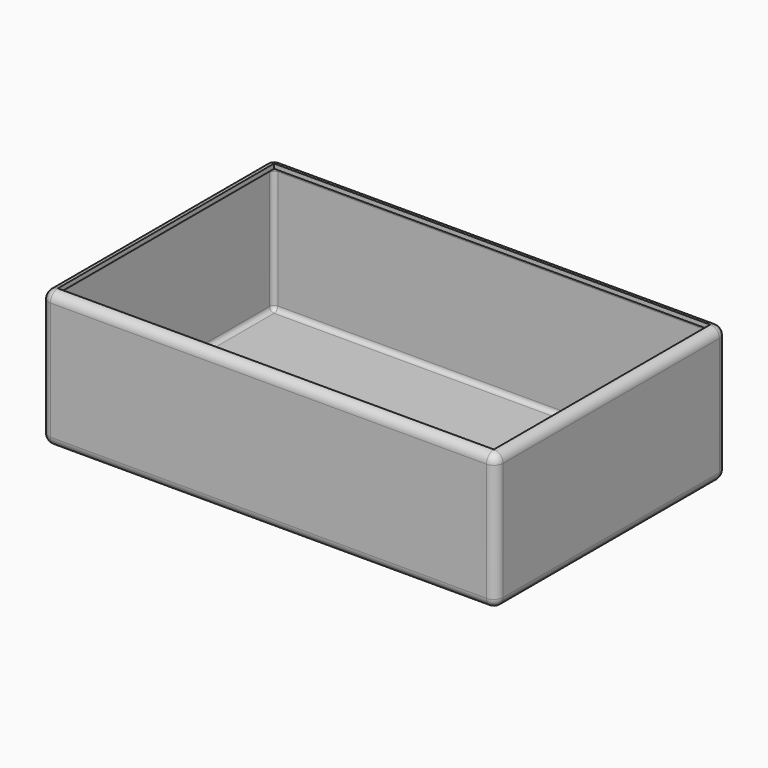
from build123d import *

# Parameters (mm, degrees)
F0_W     = 155.229896307
F0_H     = 82.4026092887
F1_DEPTH = 75.438
F2_DEPTH = 77.216
F3_DEPTH = 96.012
F4_R     = 5.08
F5_T     = -2.54
F6_R     = 16.8009840587
F7_DEPTH = 2.54


# Not quite as in the source:
# - a shell that OpenCascade refuses in one call is made with other operations: the cavity is built on its own and cut out


with BuildPart() as f1:
    # F0 (on Top) → F1 (new body)
    with BuildSketch(Plane.XY):
        with Locations((77.6149481535, 41.2013046443)):
            Rectangle(F0_W, F0_H)
    extrude(amount=F1_DEPTH)

    # F2 (add): a face of the model
    f2_faces = [f1.faces().sort_by_distance(p)[0] for p in [
        (77.6149481535, 0, 37.719),
    ]]
    extrude(f2_faces, amount=F2_DEPTH)

    # F3 (add): a face of the model
    f3_faces = [f1.faces().sort_by_distance(p)[0] for p in [
        (0, 2.5933046443, 37.719),
    ]]
    extrude(f3_faces, amount=F3_DEPTH)

    # F4
    f4_edges = [f1.edges().sort_by_distance(p)[0] for p in [
        (-96.012, 2.593305, 75.438),
        (29.608948, -77.216, 75.438),
        (29.608948, -77.216, 0),
        (-96.012, -77.216, 37.719),
        (-96.012, 2.593305, 0),
        (29.608948, 82.402609, 75.438),
        (155.229896, 2.593305, 75.438),
        (155.229896, -77.216, 37.719),
        (-96.012, 82.402609, 37.719),
        (29.608948, 82.402609, 0),
        (155.229896, 82.402609, 37.719),
        (155.229896, 2.593305, 0),
    ]]
    fillet(f4_edges, radius=F4_R)

    # F5: a shell. OpenCascade refuses it in one call, so the cavity is built on its own and cut out:
    # the body offset inwards by the wall thickness, plus a prism from it out through each open face.
    f5_core = offset(f1.part, amount=F5_T, mode=Mode.PRIVATE)
    f5_exits = [f5_core.faces().sort_by_distance(p)[0] for p in [
        (29.608948, 2.593305, 72.898),
    ]]
    add(f5_core, mode=Mode.SUBTRACT)
    extrude(f5_exits, amount=-F5_T, mode=Mode.SUBTRACT)

    # F6 (on face) → F7 (join, through all)
    with BuildSketch(Plane.YZ.offset(155.229896307)):
        with Locations((0, 37.719)):
            Circle(F6_R)
    extrude(amount=-F7_DEPTH)


solid = f1.part
